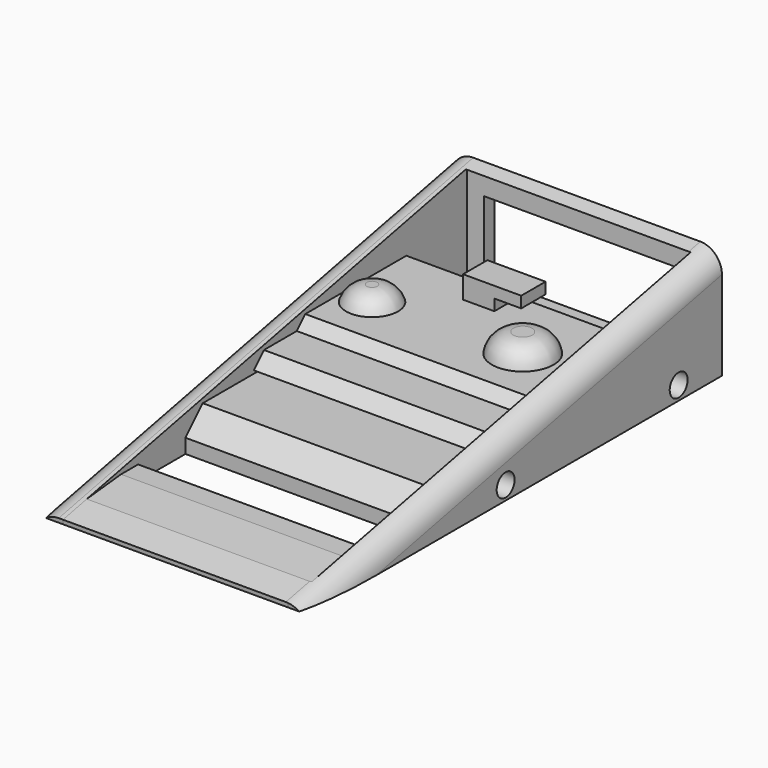
from build123d import *

# Parameters (mm, degrees)
F1_DEPTH      = 31.75
F2_W          = 52.7695193887
F2_H          = 120.6567846239
F3_DEPTH      = 25.4
F4_W          = 44.4975402206
F4_H          = 18.5406431556
F5_DEPTH      = 25.4
F6_W          = 34.7439497709
F6_H          = 5.4911417693
F7_DEPTH      = 54.31181
F8_W          = 12.1364339493
F8_H          = 2.9900523731
F9_DEPTH      = 56.69838
F10_W         = 22.7860264232
F10_H         = 8.4337261604
F11_DEPTH     = 56.06512
F12_T1_DEPTH  = 52.7695193887
F12_T6_DEPTH  = 52.7695193887
F12_T11_DEPTH = 52.7695193887
F14_DEPTH     = 55.98348
F15_T1_DEPTH  = 52.7695193887
F16_R         = 7.2468545108
F17_DEPTH     = 4.48168
F19_SIZE      = 5.08
F20_T1_DEPTH  = 149.6281885647
F21_R         = 6.1019617507
F22_DEPTH     = 3.60881
F24_R         = 2.6289
F25_DEPTH     = 82.93478
F26_DEPTH     = 96.11065
F27_W         = 7.3527656496
F27_H         = 7.1394555271
F28_DEPTH     = 1.80312
F29_DEPTH     = 3.46127
F30_W         = 7.1394555271
F30_H         = 2.632195
F31_DEPTH     = 6.31406


# Not quite as in the source:
# - a fillet or chamfer that OpenCascade refuses, or shapes differently, is made with other operations: its cross-section is extruded or revolved along the edge and cut away or added


with BuildPart() as f1:
    # F0 (on Right) → F1 (new body, symmetric)
    with BuildSketch(Plane.YZ):
        Polygon((55.6219257414, 26.0995179415), (-71.0249170661, 0), (55.6219257414, 0), align=None)
    extrude(amount=F1_DEPTH, both=True)

    # F2 (on face) → F3 (cut)
    with BuildSketch(Plane(origin=(0, 0, 0), x_dir=(1, 0, 0), z_dir=(0, 0, -1))):
        with Locations((0.7131025195, 7.7014956623)):
            Rectangle(F2_W, F2_H)
    extrude(amount=-F3_DEPTH, mode=Mode.SUBTRACT)

    # F4 (on face) → F5 (cut)
    with BuildSketch(Plane.XZ.offset(-52.6268966496)):
        with Locations((0.5704807118, 11.6948671639)):
            Rectangle(F4_W, F4_H)
    extrude(amount=-F5_DEPTH, mode=Mode.SUBTRACT)

    # F6 (on face) → F7 (join)
    with BuildSketch(Plane.YZ.offset(-25.6716571748)):
        with Locations((17.3719748855, 11.8913206175)):
            Rectangle(F6_W, F6_H)
    extrude(amount=F7_DEPTH)

    # F8 (on face) → F9 (join)
    with BuildSketch(Plane.YZ.offset(-25.6716571748)):
        with Locations((-6.0682169747, 10.6407759194)):
            Rectangle(F8_W, F8_H)
    extrude(amount=F9_DEPTH)

    # F10 (on face) → F11 (join)
    with BuildSketch(Plane.YZ.offset(-25.6716571748)):
        with Locations((-18.7075927729, 4.2168630802)):
            Rectangle(F10_W, F10_H)
    extrude(amount=F11_DEPTH)

    # F12: chamfer of 5.08 on 3 edges, made by hand

    # F12_s2 → F12_t1 (cut)
    with BuildSketch(Plane.YZ.offset(-25.6716571748)):
        Polygon((-30.1006059845, 3.3537261604), (-25.0206059845, 8.4337261604), (-30.1006059845, 8.4337261604), align=None)
    extrude(amount=F12_T1_DEPTH, mode=Mode.SUBTRACT)


with BuildPart() as f12_tool4:
    # F12_s5 → F12_t6 (new body)
    with BuildSketch(Plane.YZ.offset(-25.6716571748)):
        Polygon((5.08, 14.6368915021), (0, 9.5568915021), (0, 14.6368915021), align=None)
    extrude(amount=F12_T6_DEPTH)

    split(bisect_by=Plane.XY.offset(12.1358021059), keep=Keep.TOP)


with BuildPart() as f1_1:
    add(f1.part)

    # F12_t3: cut F12_tool4
    add(f12_tool4.part, mode=Mode.SUBTRACT)


with BuildPart() as f12_tool9:
    # F12_s10 → F12_t11 (new body)
    with BuildSketch(Plane.YZ.offset(-25.6716571748)):
        Polygon((-12.1364339493, 7.0558021059), (-7.0564339493, 12.1358021059), (-12.1364339493, 12.1358021059), align=None)
    extrude(amount=F12_T11_DEPTH)

    split(bisect_by=Plane.XY.offset(8.4337261604), keep=Keep.TOP)


with BuildPart() as f1_2:
    add(f1_1.part)

    # F12_t8: cut F12_tool9
    add(f12_tool9.part, mode=Mode.SUBTRACT)

    # F13 (on face) → F14 (join)
    with BuildSketch(Plane.YZ.offset(-25.6716571748)):
        Polygon((-68.0298879743, 0), (-44.0034680068, 0), (-44.0034680068, 3.4875369165), (-54.1017868902, 3.4875369165), (-68.0298879743, 0.6172188251), align=None)
    extrude(amount=F14_DEPTH)

    # F15: chamfer of 5.08 on 1 edges, made by hand

    # F15_s2 → F15_t1 (cut)
    with BuildSketch(Plane.YZ.offset(-25.6716571748)):
        with BuildLine():
            Line((-59.2793850519, 2.4415783127), (-48.81963513, 3.5081501604))
            Line((-48.81963513, 3.5081501604), (-48.81963513, 3.6097501604))
            ThreePointArc((-48.81963513, 3.6097501604), (-51.4607110101, 3.5891369165), (-54.1017868902, 3.5891369165))
            Line((-54.1017868902, 3.5891369165), (-54.1222937974, 3.5870458445))
            ThreePointArc((-54.1222937974, 3.5870458445), (-56.7090125934, 3.0539720456), (-59.2998919591, 2.5410872407))
            Line((-59.2998919591, 2.5410872407), (-59.2793850519, 2.4415783127))
        make_face()
    extrude(amount=F15_T1_DEPTH, mode=Mode.SUBTRACT)

    # F16 (on face) → F17 (join)
    with BuildSketch(Plane.XY.offset(14.6368915021)):
        with Locations((15.2392005548, 17.7897959948)):
            Circle(F16_R)
    extrude(amount=F17_DEPTH)

    # F18: fillet of radius 5.08 on 1 edges, made by hand

    # F18_s1 → F18_t2 (revolve, cut)
    with BuildSketch(Plane.XZ.offset(-17.7897959948)):
        with BuildLine():
            ThreePointArc((22.4860550656, 14.6368915021), (20.8153524575, 17.8363251539), (17.4414130389, 19.1185715021))
            Line((17.4414130389, 19.1185715021), (22.4860550656, 19.1185715021))
            Line((22.4860550656, 19.1185715021), (22.4860550656, 14.6368915021))
        make_face()
    revolve(axis=Axis((15.2392005548, 17.7897959948, 19.1185715021), (0, 0, 1)), mode=Mode.SUBTRACT)

    # F19
    f19_edges = [f1_2.edges().sort_by_distance(p)[0] for p in [
        (0, -71.024917, 0),
    ]]
    chamfer(f19_edges, length=F19_SIZE)

    # F20: fillet of radius 5.08 on 2 edges, made by hand

    # F20_s2 → F20_t1 (cut)
    with BuildSketch(Plane(origin=(0, 70.954042843, 14.6222856658), x_dir=(1, 0, 0), z_dir=(0, -0.9794185829, -0.2018396378))):
        with BuildLine():
            ThreePointArc((-26.67, 14.3356435337), (-30.2621024484, 12.8477459822), (-31.75, 9.2556435337))
            Line((-31.75, 9.2556435337), (-31.75, 14.3356435337))
            Line((-31.75, 14.3356435337), (-26.67, 14.3356435337))
        make_face()
        with BuildLine():
            ThreePointArc((26.67, 14.3356435337), (30.2621024484, 12.8477459822), (31.75, 9.2556435337))
            Line((31.75, 9.2556435337), (31.75, 14.3356435337))
            Line((31.75, 14.3356435337), (26.67, 14.3356435337))
        make_face()
    extrude(amount=F20_T1_DEPTH, mode=Mode.SUBTRACT)

    # F21 (on face) → F22 (join)
    with BuildSketch(Plane.XY.offset(14.6368915021)):
        with Locations((-19.1379822791, 16.5131352842)):
            Circle(F21_R)
    extrude(amount=F22_DEPTH)

    # F23: fillet of radius 5.08 on 1 edges, made by hand

    # F23_s1 → F23_t2 (revolve, cut)
    with BuildSketch(Plane.XZ.offset(-16.5131352842)):
        with BuildLine():
            ThreePointArc((-13.0360205283, 14.6368915021), (-14.8707219244, 17.2449198831), (-17.8983245073, 18.2457015021))
            Line((-17.8983245073, 18.2457015021), (-13.0360205283, 18.2457015021))
            Line((-13.0360205283, 18.2457015021), (-13.0360205283, 14.6368915021))
        make_face()
    revolve(axis=Axis((-19.1379822791, 16.5131352842, 18.2457015021), (0, 0, 1)), mode=Mode.SUBTRACT)

    # F24 (on face) → F25 (cut)
    with BuildSketch(Plane.YZ.offset(31.75)):
        with Locations((-7.8780742586, 3.2512)):
            Circle(F24_R)
    extrude(amount=-F25_DEPTH, mode=Mode.SUBTRACT)

    # F24 (on face) → F26 (cut, symmetric)
    with BuildSketch(Plane.YZ.offset(31.75)):
        with Locations((-7.8780742586, 3.2512)):
            Circle(F24_R)
        with Locations((42.9219257414, 3.2512)):
            Circle(F24_R)
    extrude(amount=F26_DEPTH, both=True, mode=Mode.SUBTRACT)

    # F27 (on face) → F28 (join)
    with BuildSketch(Plane.XY.offset(14.6368915021)):
        with Locations((-2.9632803053, 31.1742220074)):
            Rectangle(F27_W, F27_H)
    extrude(amount=F28_DEPTH)

    # F29 (add): a face of the model
    f29_faces = [f1_2.faces().sort_by_distance(p)[0] for p in [
        (-2.9632803053, 31.1742220074, 16.4400115021),
    ]]
    extrude(f29_faces, amount=F29_DEPTH)

    # F30 (on face) → F31 (join)
    with BuildSketch(Plane.YZ.offset(0.7131025195)):
        with Locations((31.1742220074, 18.5851840021)):
            Rectangle(F30_W, F30_H)
    extrude(amount=F31_DEPTH)


solid = f1_2.part
